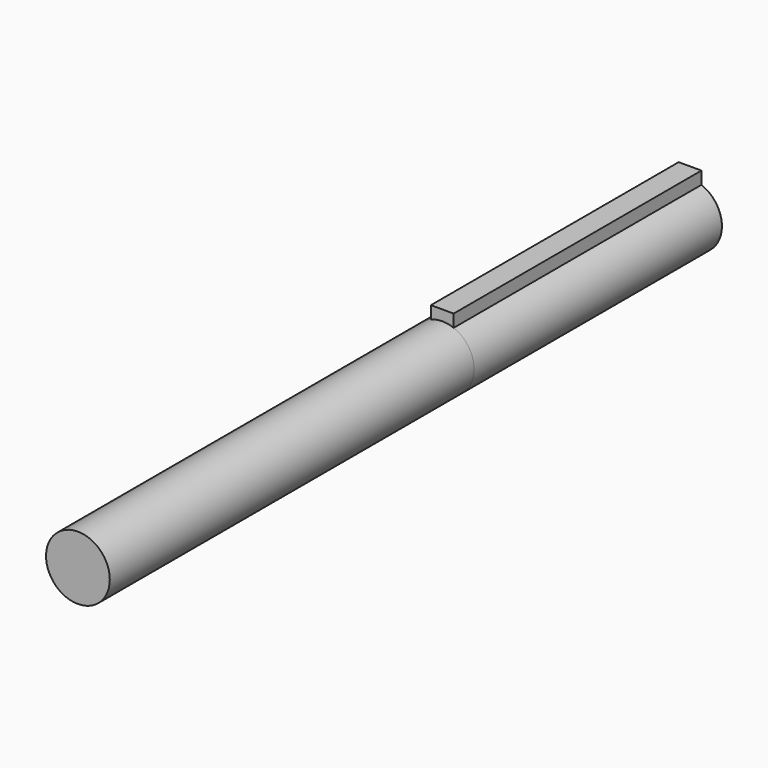
from build123d import *
from build123d import SkipClean  # not in build123d's __all__

# Parameters (mm, degrees)
F1_DEPTH = 34
F2_R     = 7
F4_DEPTH = 100


with BuildPart() as f1:
    # F0 (on Front) → F1 (new body, symmetric)
    with BuildSketch(Plane.XZ):
        with BuildLine():
            Line((2.5, 9.2983484153), (-2.5, 9.2983484153))
            Line((-2.5, 9.2983484153), (-2.5, 6.5383484153))
            ThreePointArc((-2.5, 6.5383484153), (0, -7), (2.5, 6.5383484153))
            Line((2.5, 6.5383484153), (2.5, 9.2983484153))
        make_face()
    extrude(amount=F1_DEPTH, both=True)

    # F2 (on face) → F4 (join)
    with BuildSketch(Plane.XZ.offset(34)):
        Circle(F2_R)
    with SkipClean():  # cleaning this boolean's faces spoils the solid; the shape is the same uncleaned
        extrude(amount=F4_DEPTH)


solid = f1.part
